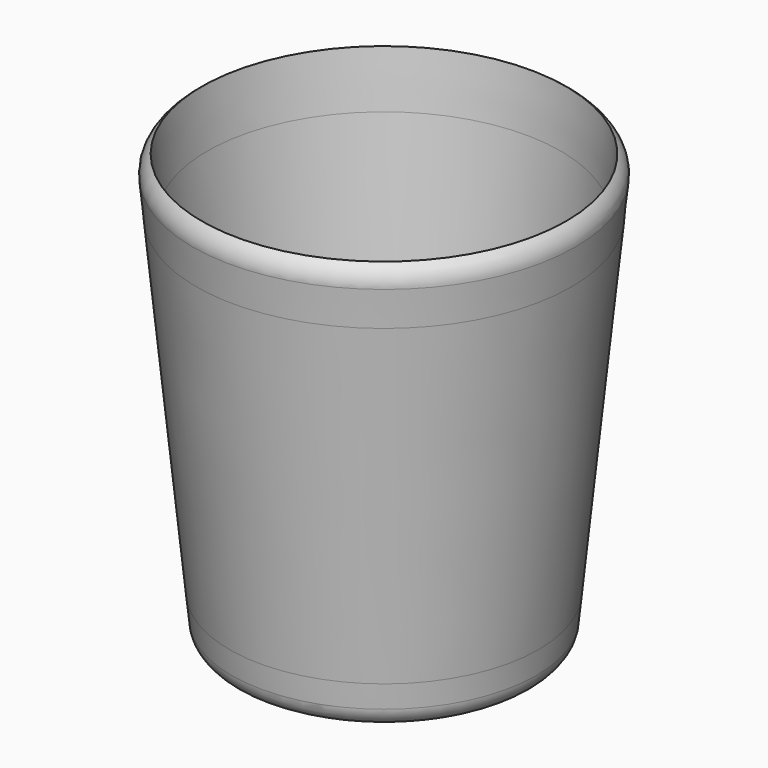
from build123d import *

# Parameters (mm, degrees)
F2_T = -2.54


# Not quite as in the source:
# - a fillet or chamfer that OpenCascade refuses, or shapes differently, is made with other operations: its cross-section is extruded or revolved along the edge and cut away or added
# - the program builds the solid bodies; features that only make, move or delete a surface that nothing else refers to are left out


with BuildPart() as f1:
    # F0 (on Front) → F1 (revolve)
    with BuildSketch(Plane.XZ):
        Polygon((39.6217921842, 43.7875076047), (-5.3782078158, 43.7875076047), (-5.3782078158, -56.2124923953), (29.6217921842, -56.2124923953), (30.6275011268, -46.1554029698), (38.3154473181, 30.724058944), align=None)
    revolve(axis=Axis((-5.3782078158, 0, -6.2124923953), (0, 0, -1)))

    # F2
    f2_openings = [f1.faces().sort_by_distance(p)[0] for p in [
        (-5.378208, 0, 43.787508),
    ]]
    offset(amount=F2_T, openings=f2_openings, kind=Kind.INTERSECTION)

    # F3: fillet of radius 5.08 on 3 edges, made by hand

    # F3_s1 → F3_t2 (revolve, cut)
    with BuildSketch(Plane.XZ):
        with BuildLine():
            ThreePointArc((30.079244295, -51.6379712879), (28.4331623981, -54.8990712658), (25.0244553687, -56.2124923953))
            Line((25.0244553687, -56.2124923953), (29.6217921842, -56.2124923953))
            Line((29.6217921842, -56.2124923953), (30.079244295, -51.6379712879))
        make_face()
    revolve(axis=Axis((-5.3782078158, 0, -56.2124923953), (0, 0, -1)), mode=Mode.SUBTRACT)

    # F3_s3 → F3_t4 (revolve, cut)
    with BuildSketch(Plane.XZ):
        with BuildLine():
            ThreePointArc((39.1587606775, 39.1571925375), (38.7342868185, 41.7523083311), (37.0691237764, 43.7875076047))
            Line((37.0691237764, 43.7875076047), (39.6217921842, 43.7875076047))
            Line((39.6217921842, 43.7875076047), (39.1587606775, 39.1571925375))
        make_face()
    revolve(axis=Axis((-5.3782078158, 0, 43.7875076047), (0, 0, -1)), mode=Mode.SUBTRACT)


solid = f1.part
